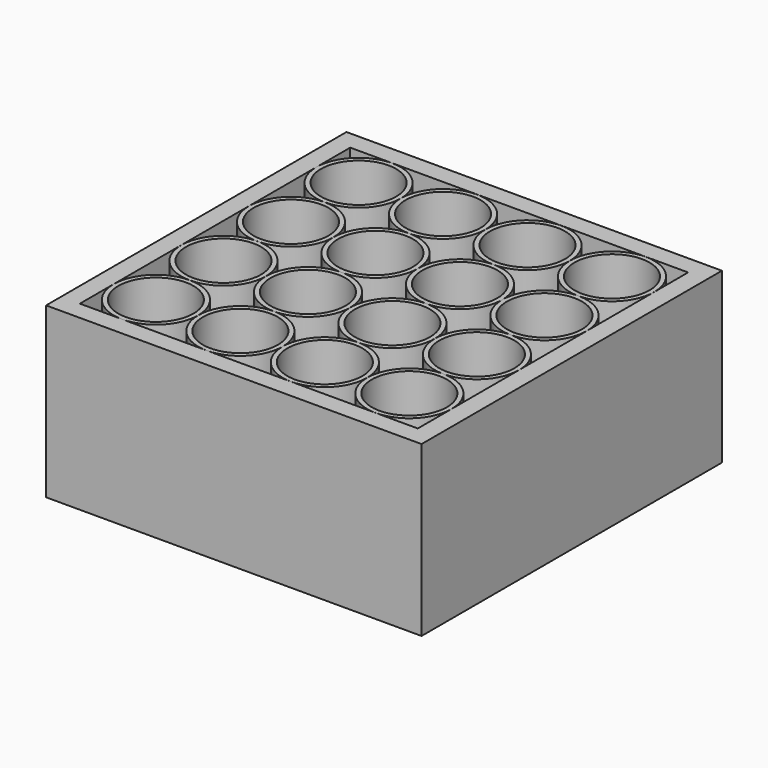
from build123d import *

# Parameters (mm, degrees)
F0_W     = 91.44
F0_H     = 91.44
F1_DEPTH = 45.72
F2_W     = 91.44
F2_H     = 91.44
F3_DEPTH = 5.08
F4_R     = 10.16
F5_DEPTH = 40.64


# Not quite as in the source:
# - ends of sketch curves that miss each other by under 0.0002 mm in the source are joined


with BuildPart() as f1:
    # F0 (on Top) → F1 (new body)
    with BuildSketch(Plane.XY):
        Polygon((96.52, 5.08), (0, 5.08), (-5.08, 5.08), (-5.08, -96.52), (96.52, -96.52), align=None)
        with Locations((45.72, -45.72)):
            Rectangle(F0_W, F0_H, mode=Mode.SUBTRACT)
    extrude(amount=F1_DEPTH)

    # F2 (on Top) → F3 (join)
    with BuildSketch(Plane.XY):
        with Locations((45.72, -45.72)):
            Rectangle(F2_W, F2_H)
    extrude(amount=F3_DEPTH)


with BuildPart() as f5:
    # F4 (on face) → F5 (new body)
    with BuildSketch(Plane.XY.offset(5.08)):
        with BuildLine():
            ThreePointArc((0, -11.4595933233), (3.3479891479, -19.5420434832), (11.4306212751, -22.8895933064))
            ThreePointArc((11.4306212751, -22.8895933064), (19.5124501599, -19.5416041754), (22.86, -11.4595933233))
            ThreePointArc((22.86, -11.4595933233), (11.43, -0.0295933233), (0, -11.4595933233))
        make_face()
        with Locations((11.43, -11.4595933233)):
            Circle(F4_R, mode=Mode.SUBTRACT)
    extrude(amount=F5_DEPTH)


with BuildPart() as f5b:
    # F4 (on face) → F5, piece 2 (new body)
    with BuildSketch(Plane.XY.offset(5.08)):
        with BuildLine():
            ThreePointArc((45.7177762473, -11.2341381352), (34.1772669227, -0.030149275), (22.86, -11.4595933233))
            ThreePointArc((22.86, -11.4595933233), (26.0970572413, -19.4295738096), (33.9747137275, -22.8852440516))
            Line((33.9747137275, -22.8852440516), (34.6052862725, -22.8852440516))
            ThreePointArc((34.6052862725, -22.8852440516), (42.4049676217, -19.5089535773), (45.7178336, -11.682122448))
            Line((45.7178336, -11.682122448), (45.7177762473, -11.2341381352))
        make_face()
        with Locations((34.29, -11.4595933233)):
            Circle(F4_R, mode=Mode.SUBTRACT)
    extrude(amount=F5_DEPTH)


with BuildPart() as f5c:
    # F4 (on face) → F5, piece 3 (new body)
    with BuildSketch(Plane.XY.offset(5.08)):
        with BuildLine():
            ThreePointArc((68.579999983, -11.4604759586), (57.1504413006, -0.0304759671), (45.720000017, -11.4595933233))
            ThreePointArc((45.720000017, -11.4595933233), (48.9461162057, -19.419193881), (56.8042052173, -22.8852440516))
            Line((56.8042052173, -22.8852440516), (56.9658252491, -22.8852440516))
            ThreePointArc((56.9658252491, -22.8852440516), (57.1512422707, -22.8837400388), (57.3366592922, -22.8852440516))
            Line((57.3366592922, -22.8852440516), (57.4957947486, -22.8852440516))
            ThreePointArc((57.4957947486, -22.8852440516), (65.3535764643, -19.4195106309), (68.579999983, -11.4604759586))
        make_face()
        with Locations((57.149999983, -11.4604759586)):
            Circle(F4_R, mode=Mode.SUBTRACT)
    extrude(amount=F5_DEPTH)


with BuildPart() as f5d:
    # F4 (on face) → F5, piece 4 (new body)
    with BuildSketch(Plane.XY.offset(5.08)):
        with BuildLine():
            ThreePointArc((80.409883046, -22.8852440516), (88.2323950704, -19.4018330263), (91.4399999148, -11.4622412292))
            ThreePointArc((91.4399999148, -11.4622412292), (80.0108825501, -0.0322412633), (68.5800000511, -11.4604759586))
            ThreePointArc((68.5800000511, -11.4604759586), (71.786991681, -19.4011980616), (79.6101167836, -22.8852440516))
            Line((79.6101167836, -22.8852440516), (79.6485893705, -22.8852440516))
            ThreePointArc((79.6485893705, -22.8852440516), (80.0112418755, -22.8794894604), (80.3738943806, -22.8852440516))
            Line((80.3738943806, -22.8852440516), (80.409883046, -22.8852440516))
        make_face()
        with Locations((80.0099999148, -11.4622412292)):
            Circle(F4_R, mode=Mode.SUBTRACT)
    extrude(amount=F5_DEPTH)


with BuildPart() as f5e:
    # F4 (on face) → F5, piece 5 (new body)
    with BuildSketch(Plane.XY.offset(5.08)):
        with BuildLine():
            ThreePointArc((11.4306212751, -22.8895933064), (0.0049345094, -34.0291071653), (10.8498374826, -45.7347966616))
            ThreePointArc((10.8498374826, -45.7347966616), (11.4312426539, -45.7200000338), (12.0126478252, -45.7347966616))
            ThreePointArc((12.0126478252, -45.7347966616), (19.7164813682, -42.1935833483), (22.8612426539, -34.3195932895))
            ThreePointArc((22.8612426539, -34.3195932895), (19.5132534693, -26.237143093), (11.4306212751, -22.8895933064))
        make_face()
        with Locations((11.4312426539, -34.3195932895)):
            Circle(F4_R, mode=Mode.SUBTRACT)
    extrude(amount=F5_DEPTH)


with BuildPart() as f5f:
    # F4 (on face) → F5, piece 6 (new body)
    with BuildSketch(Plane.XY.offset(5.08)):
        with BuildLine():
            ThreePointArc((22.861242789, -34.3195932895), (26.0244845177, -42.210498391), (33.7608792372, -45.7347966616))
            ThreePointArc((33.7608792372, -45.7347966616), (34.2912425188, -45.7224853415), (34.8216058003, -45.7347966616))
            ThreePointArc((34.8216058003, -45.7347966616), (42.4810469796, -42.2903132904), (45.7190432097, -34.5413207567))
            Line((45.7190432097, -34.5413207567), (45.7189764797, -34.0933364523))
            ThreePointArc((45.7189764797, -34.0933364523), (42.3536988309, -26.2151515382), (34.4591606398, -22.8883414909))
            ThreePointArc((34.4591606398, -22.8883414909), (34.2906213269, -22.8895933064), (34.1220818789, -22.8883598142))
            ThreePointArc((34.1220818789, -22.8883598142), (26.1485522378, -26.2957929407), (22.861242789, -34.3195932895))
        make_face()
        with Locations((34.2912425188, -34.3171079818)):
            Circle(F4_R, mode=Mode.SUBTRACT)
    extrude(amount=F5_DEPTH)


with BuildPart() as f5g:
    # F4 (on face) → F5, piece 7 (new body)
    with BuildSketch(Plane.XY.offset(5.08)):
        with BuildLine():
            ThreePointArc((45.7212427669, -34.3171079817), (48.9118984459, -42.2357418904), (56.699174115, -45.7347966616))
            ThreePointArc((56.699174115, -45.7347966616), (56.7769181976, -45.7319843476), (56.8546796205, -45.7297012378))
            ThreePointArc((56.8546796205, -45.7297012378), (57.1529262422, -45.7258534086), (57.4511717171, -45.7297891184))
            Line((57.4511717171, -45.7297891184), (57.7150116349, -45.7298279897))
            ThreePointArc((57.7150116349, -45.7298279897), (65.4303963287, -42.194127598), (68.5812422707, -34.3137400388))
            ThreePointArc((68.5812422707, -34.3137400388), (65.3307618548, -26.3299840698), (57.4280735266, -22.8870929166))
            ThreePointArc((57.4280735266, -22.8870929166), (57.1506213099, -22.8904759417), (56.873168727, -22.8871230808))
            ThreePointArc((56.873168727, -22.8871230808), (48.9701126219, -26.3316339464), (45.7212427669, -34.3171079817))
        make_face()
        with Locations((57.1512422707, -34.3137400388)):
            Circle(F4_R, mode=Mode.SUBTRACT)
    extrude(amount=F5_DEPTH)


with BuildPart() as f5h:
    # F4 (on face) → F5, piece 8 (new body)
    with BuildSketch(Plane.XY.offset(5.08)):
        with BuildLine():
            ThreePointArc((91.44, -34.1410028682), (88.1683148887, -26.3028010153), (80.3923428869, -22.8858445947))
            ThreePointArc((80.3923428869, -22.8858445947), (80.0106212417, -22.8922412123), (79.6288989034, -22.885886095))
            ThreePointArc((79.6288989034, -22.885886095), (71.7934673353, -26.3651152493), (68.5812426659, -34.3137400386))
            ThreePointArc((68.5812426659, -34.3137400386), (71.7960440402, -42.2565281874), (79.6278116032, -45.7330563826))
            Line((79.6278116032, -45.7330563826), (79.7506664615, -45.7330744827))
            ThreePointArc((79.7506664615, -45.7330744827), (80.012925847, -45.7301039869), (80.2751843459, -45.7331517595))
            Line((80.2751843459, -45.7331517595), (80.3913060838, -45.7331688676))
            ThreePointArc((80.3913060838, -45.7331688676), (88.1679515398, -42.3165480623), (91.44, -34.4779760527))
            Line((91.44, -34.4779760527), (91.44, -34.1410028682))
        make_face()
        with Locations((80.0112418755, -34.3094894604)):
            Circle(F4_R, mode=Mode.SUBTRACT)
    extrude(amount=F5_DEPTH)


with BuildPart() as f5i:
    # F4 (on face) → F5, piece 9 (new body)
    with BuildSketch(Plane.XY.offset(5.08)):
        with BuildLine():
            ThreePointArc((68.5812426659, -57.1558532847), (71.7934673353, -65.1044780739), (79.6288989034, -68.5837072283))
            ThreePointArc((79.6288989034, -68.5837072283), (80.0106212417, -68.577352111), (80.3923428869, -68.5837487286))
            ThreePointArc((80.3923428869, -68.5837487286), (88.1683148887, -65.1667923079), (91.44, -57.3285904551))
            Line((91.44, -57.3285904551), (91.44, -56.9916172706))
            ThreePointArc((91.44, -56.9916172706), (88.1495092479, -49.1343014621), (80.3387405139, -45.7347966616))
            ThreePointArc((80.3387405139, -45.7347966616), (80.0112418755, -45.7394894604), (79.6837432371, -45.7347966616))
            ThreePointArc((79.6837432371, -45.7347966616), (71.815522108, -49.1929790683), (68.5812426659, -57.1558532847))
        make_face()
        with Locations((80.0112418755, -57.1601038628)):
            Circle(F4_R, mode=Mode.SUBTRACT)
    extrude(amount=F5_DEPTH)


with BuildPart() as f5j:
    # F4 (on face) → F5, piece 10 (new body)
    with BuildSketch(Plane.XY.offset(5.08)):
        with BuildLine():
            ThreePointArc((45.7212427669, -57.1524853415), (48.9701126219, -65.1379593769), (56.873168727, -68.5824702425))
            ThreePointArc((56.873168727, -68.5824702425), (57.1506213099, -68.5791173816), (57.4280735266, -68.5825004067))
            ThreePointArc((57.4280735266, -68.5825004067), (65.3307618548, -65.1396092535), (68.5812422707, -57.1558532845))
            ThreePointArc((68.5812422707, -57.1558532845), (65.3917531474, -49.2350654139), (57.6033104263, -45.7347966616))
            ThreePointArc((57.6033104263, -45.7347966616), (57.1512422707, -45.7437400388), (56.699174115, -45.7347966616))
            ThreePointArc((56.699174115, -45.7347966616), (48.9118984459, -49.2338514329), (45.7212427669, -57.1524853415))
        make_face()
        with Locations((57.1512422707, -57.1558532845)):
            Circle(F4_R, mode=Mode.SUBTRACT)
    extrude(amount=F5_DEPTH)


with BuildPart() as f5k:
    # F4 (on face) → F5, piece 11 (new body)
    with BuildSketch(Plane.XY.offset(5.08)):
        with BuildLine():
            ThreePointArc((22.861242789, -57.1500000338), (26.1485522378, -65.1738003826), (34.1220818789, -68.5812335091))
            ThreePointArc((34.1220818789, -68.5812335091), (34.2906213269, -68.5800000169), (34.4591606398, -68.5812518324))
            ThreePointArc((34.4591606398, -68.5812518324), (42.3536988309, -65.2544417851), (45.7190518581, -57.3762568835))
            Line((45.7190518581, -57.3762568835), (45.7189764797, -56.9282725763))
            ThreePointArc((45.7189764797, -56.9282725763), (42.4810469796, -49.1792800328), (34.8216058003, -45.7347966616))
            ThreePointArc((34.8216058003, -45.7347966616), (34.2912425188, -45.7471079818), (33.7608792372, -45.7347966616))
            ThreePointArc((33.7608792372, -45.7347966616), (26.0244845177, -49.2590949322), (22.861242789, -57.1500000338))
        make_face()
        with Locations((34.2912425188, -57.1524853415)):
            Circle(F4_R, mode=Mode.SUBTRACT)
    extrude(amount=F5_DEPTH)


with BuildPart() as f5l:
    # F4 (on face) → F5, piece 12 (new body)
    with BuildSketch(Plane.XY.offset(5.08)):
        with BuildLine():
            ThreePointArc((10.8498374826, -45.7347966616), (0.0049345109, -57.4404862164), (11.4306213921, -68.5800000169))
            ThreePointArc((11.4306213921, -68.5800000169), (19.5132535107, -65.2324501889), (22.8612426539, -57.1500000338))
            ThreePointArc((22.8612426539, -57.1500000338), (19.7164813682, -49.276009975), (12.0126478252, -45.7347966616))
            ThreePointArc((12.0126478252, -45.7347966616), (11.4312426539, -45.7495932895), (10.8498374826, -45.7347966616))
        make_face()
        with Locations((11.4312426539, -57.1500000338)):
            Circle(F4_R, mode=Mode.SUBTRACT)
    extrude(amount=F5_DEPTH)


with BuildPart() as f5m:
    # F4 (on face) → F5, piece 13 (new body)
    with BuildSketch(Plane.XY.offset(5.08)):
        with BuildLine():
            ThreePointArc((11.4306213921, -68.5800000169), (3.3479891893, -71.9275497987), (0, -80.01))
            ThreePointArc((0, -80.01), (3.347769491, -88.092230509), (11.43, -91.44))
            ThreePointArc((11.43, -91.44), (19.512230509, -88.092230509), (22.86, -80.01))
            ThreePointArc((22.86, -80.01), (19.5124502013, -71.9279891893), (11.4306213921, -68.5800000169))
        make_face()
        with Locations((11.43, -80.01)):
            Circle(F4_R, mode=Mode.SUBTRACT)
    extrude(amount=F5_DEPTH)


with BuildPart() as f5n:
    # F4 (on face) → F5, piece 14 (new body)
    with BuildSketch(Plane.XY.offset(5.08)):
        with BuildLine():
            ThreePointArc((33.9747137275, -68.5843492716), (26.0970572413, -72.0400195137), (22.86, -80.01))
            ThreePointArc((22.86, -80.01), (26.207769491, -88.092230509), (34.29, -91.44))
            ThreePointArc((34.29, -91.44), (42.2921230683, -88.1715517152), (45.7177762473, -80.235455188))
            Line((45.7177762473, -80.235455188), (45.7177582215, -79.7874708796))
            ThreePointArc((45.7177582215, -79.7874708796), (42.4049676217, -71.960639746), (34.6052862725, -68.5843492716))
            Line((34.6052862725, -68.5843492716), (33.9747137275, -68.5843492716))
        make_face()
        with Locations((34.29, -80.01)):
            Circle(F4_R, mode=Mode.SUBTRACT)
    extrude(amount=F5_DEPTH)


with BuildPart() as f5o:
    # F4 (on face) → F5, piece 15 (new body)
    with BuildSketch(Plane.XY.offset(5.08)):
        with BuildLine():
            ThreePointArc((56.8042052173, -68.5843492716), (48.9461162057, -72.0503994423), (45.720000017, -80.01))
            ThreePointArc((45.720000017, -80.01), (57.1504413006, -91.4391173562), (68.579999983, -80.0091173647))
            ThreePointArc((68.579999983, -80.0091173647), (65.3535764643, -72.0500826924), (57.4957947486, -68.5843492716))
            Line((57.4957947486, -68.5843492716), (57.3366592922, -68.5843492716))
            ThreePointArc((57.3366592922, -68.5843492716), (57.1512422707, -68.5858532845), (56.9658252491, -68.5843492716))
            Line((56.9658252491, -68.5843492716), (56.8042052173, -68.5843492716))
        make_face()
        with Locations((57.149999983, -80.0091173647)):
            Circle(F4_R, mode=Mode.SUBTRACT)
    extrude(amount=F5_DEPTH)


with BuildPart() as f5p:
    # F4 (on face) → F5, piece 16 (new body)
    with BuildSketch(Plane.XY.offset(5.08)):
        with BuildLine():
            ThreePointArc((79.6101167836, -68.5843492716), (71.786991681, -72.0683952617), (68.5800000511, -80.0091173647))
            ThreePointArc((68.5800000511, -80.0091173647), (80.0108825501, -91.43735206), (91.4399999148, -80.0073520941))
            ThreePointArc((91.4399999148, -80.0073520941), (91.4399999063, -80.0069107764), (91.4399998807, -80.0064694588))
            ThreePointArc((91.4399998807, -80.0064694588), (88.2320885129, -72.0674428324), (80.409883046, -68.5843492716))
            Line((80.409883046, -68.5843492716), (80.3738943806, -68.5843492716))
            ThreePointArc((80.3738943806, -68.5843492716), (80.0112418755, -68.5901038628), (79.6485893705, -68.5843492716))
            Line((79.6485893705, -68.5843492716), (79.6101167836, -68.5843492716))
        make_face()
        with Locations((80.0099999148, -80.0073520941)):
            Circle(F4_R, mode=Mode.SUBTRACT)
    extrude(amount=F5_DEPTH)


solid = Compound([f1.part, f5.part, f5b.part, f5c.part, f5d.part, f5e.part, f5f.part, f5g.part, f5h.part, f5i.part, f5j.part, f5k.part, f5l.part, f5m.part, f5n.part, f5o.part, f5p.part])
